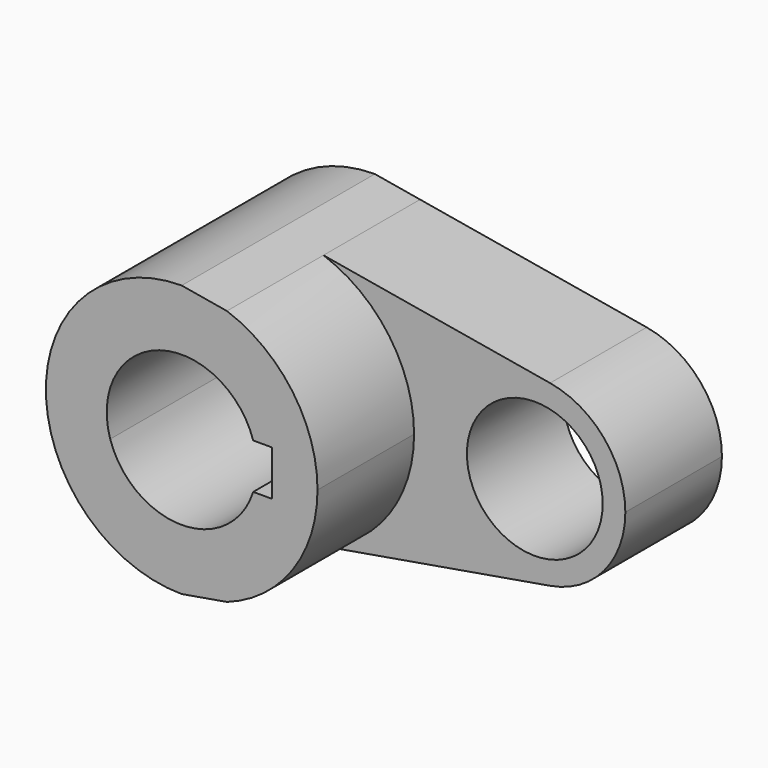
from build123d import *

# Parameters (mm, degrees)
F0_R     = 14.2875
F1_DEPTH = 25.4
F2_DEPTH = 50.8


with BuildPart() as f1:
    # F0 (on Front) → F1 (new body)
    with BuildSketch(Plane.XZ):
        with BuildLine():
            Line((9.5121844836, 26.9452959039), (0, 28.575))
            ThreePointArc((0, 28.575), (-28.575, 0), (0, -28.575))
            Line((0, -28.575), (9.5121844836, -26.9452959039))
            ThreePointArc((9.5121844836, -26.9452959039), (23.3274655355, -16.5033322905), (28.575, 0))
            ThreePointArc((28.575, 0), (23.3274655355, 16.5033322905), (9.5121844836, 26.9452959039))
        make_face()
        with BuildLine():
            ThreePointArc((-15.0423806475, 4.7625), (0, 15.778295909), (15.0423806475, 4.7625))
            Line((15.0423806475, 4.7625), (19.05, 4.7625))
            Line((19.05, 4.7625), (19.05, -4.7625))
            Line((19.05, -4.7625), (15.0423806475, -4.7625))
            ThreePointArc((15.0423806475, -4.7625), (0, -15.778295909), (-15.0423806475, -4.7625))
            Line((-15.0423806475, -4.7625), (-19.05, -4.7625))
            Line((-19.05, -4.7625), (-19.05, 4.7625))
            Line((-19.05, 4.7625), (-15.0423806475, 4.7625))
        make_face(mode=Mode.SUBTRACT)
        with BuildLine():
            Line((57.1919272622, 18.7764181619), (9.5121844836, 26.9452959039))
            ThreePointArc((9.5121844836, 26.9452959039), (23.3274655355, 16.5033322905), (28.575, 0))
            ThreePointArc((28.575, 0), (23.3274655355, -16.5033322905), (9.5121844836, -26.9452959039))
            Line((9.5121844836, -26.9452959039), (57.1919272622, -18.7764181619))
            ThreePointArc((57.1919272622, -18.7764181619), (34.925, 0), (57.1919272622, 18.7764181619))
        make_face()
        with BuildLine():
            ThreePointArc((73.025, 0), (68.5383952831, 12.2804730295), (57.1919272622, 18.7764181619))
            ThreePointArc((57.1919272622, 18.7764181619), (34.925, 0), (57.1919272622, -18.7764181619))
            ThreePointArc((57.1919272622, -18.7764181619), (68.5383952831, -12.2804730295), (73.025, 0))
        make_face()
        with Locations((53.975, 0)):
            Circle(F0_R, mode=Mode.SUBTRACT)
        with BuildLine():
            ThreePointArc((-15.0423806475, -4.7625), (-15.778295909, 0), (-15.0423806475, 4.7625))
            Line((-15.0423806475, 4.7625), (-19.05, 4.7625))
            Line((-19.05, 4.7625), (-19.05, -4.7625))
            Line((-19.05, -4.7625), (-15.0423806475, -4.7625))
        make_face()
    extrude(amount=F1_DEPTH)

    # F0 (on Front) → F2 (join)
    with BuildSketch(Plane.XZ):
        with BuildLine():
            Line((9.5121844836, 26.9452959039), (0, 28.575))
            ThreePointArc((0, 28.575), (-28.575, 0), (0, -28.575))
            Line((0, -28.575), (9.5121844836, -26.9452959039))
            ThreePointArc((9.5121844836, -26.9452959039), (23.3274655355, -16.5033322905), (28.575, 0))
            ThreePointArc((28.575, 0), (23.3274655355, 16.5033322905), (9.5121844836, 26.9452959039))
        make_face()
        with BuildLine():
            ThreePointArc((-15.0423806475, 4.7625), (0, 15.778295909), (15.0423806475, 4.7625))
            Line((15.0423806475, 4.7625), (19.05, 4.7625))
            Line((19.05, 4.7625), (19.05, -4.7625))
            Line((19.05, -4.7625), (15.0423806475, -4.7625))
            ThreePointArc((15.0423806475, -4.7625), (0, -15.778295909), (-15.0423806475, -4.7625))
            Line((-15.0423806475, -4.7625), (-19.05, -4.7625))
            Line((-19.05, -4.7625), (-19.05, 4.7625))
            Line((-19.05, 4.7625), (-15.0423806475, 4.7625))
        make_face(mode=Mode.SUBTRACT)
        with BuildLine():
            ThreePointArc((-15.0423806475, -4.7625), (-15.778295909, 0), (-15.0423806475, 4.7625))
            Line((-15.0423806475, 4.7625), (-19.05, 4.7625))
            Line((-19.05, 4.7625), (-19.05, -4.7625))
            Line((-19.05, -4.7625), (-15.0423806475, -4.7625))
        make_face()
    extrude(amount=F2_DEPTH)


solid = f1.part
